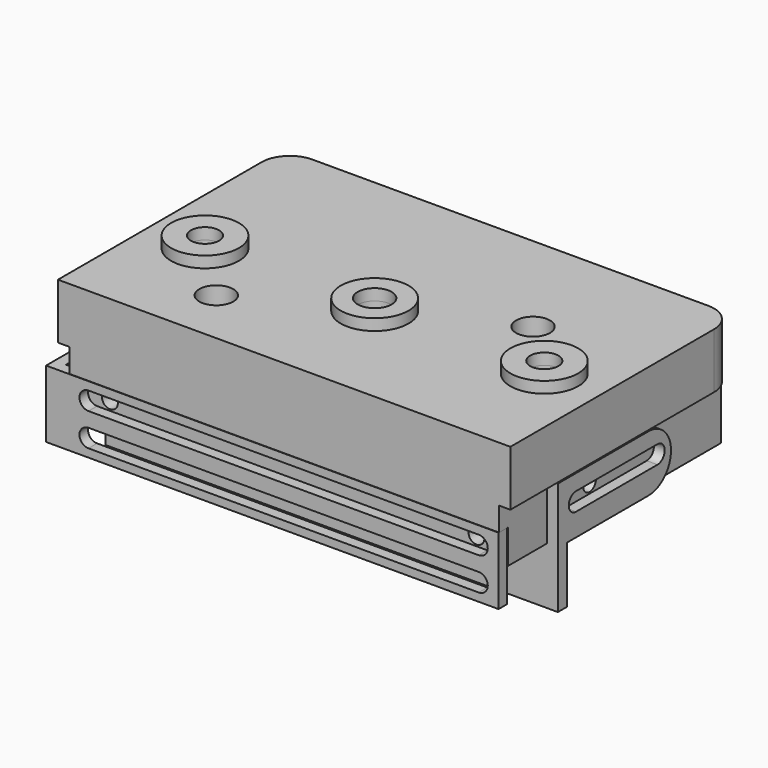
from build123d import *

# Parameters (mm, degrees)
F0_W          = 80
F0_H          = 50
F0_R          = 3
F0_R_2        = 5.1
F1_DEPTH      = 20
F3_DEPTH      = 20
F4_R          = 5
F4_R_2        = 2.5
F5_DEPTH      = 20
F5_DEPTH_BACK = 2
F4_R_3        = 3
F6_R          = 6
F6_R_2        = 5.1
F6_R_3        = 4.2549241369
F7_DEPTH      = 2
F6_R_4        = 3.9454924111
F6_R_5        = 4.3855625848
F8_W          = 80
F8_H          = 2
F9_DEPTH      = 10
F10_W         = 2
F10_H         = 50
F11_DEPTH     = 10.2
F12_W         = 1.9
F12_H         = 25
F13_DEPTH     = 10
F15_DEPTH     = 90
F16_R         = 4.99999
F17_R         = 1.4
F18_R         = 1.4
F19_DEPTH     = 2.5
F20_R         = 5
F21_W         = 2
F21_H         = 6
F22_DEPTH     = 80
F24_START     = 0.1
F23_W         = 12.5
F23_H         = 5.95
F23_W_2       = 10.5
F23_H_2       = 11.9
F24_DEPTH     = 2
F25_W         = 1.9
F25_H         = 11.9
F26_DEPTH     = 80
F27_W         = 9
F27_H         = 3
F28_DEPTH     = 25
F29_R         = 2
F31_DEPTH     = 25
F32_R         = 1.4
F33_DEPTH     = 5


# Not quite as in the source:
# - a fillet or chamfer is up to 0.001 mm smaller than in the source, because OpenCascade refuses the exact size
# - a feature names something its author has since deleted; it is built from what else it names


with BuildPart() as f1:
    # F0 (on Top) → F1 (new body)
    with BuildSketch(Plane.XY):
        Rectangle(F0_W, F0_H)
        with Locations((-20, -15)):
            Circle(F0_R, mode=Mode.SUBTRACT)
        with Locations((-30, -5)):
            Circle(F0_R_2, mode=Mode.SUBTRACT)
        with Locations((0, -5)):
            Circle(F0_R_2, mode=Mode.SUBTRACT)
        with Locations((30, -5)):
            Circle(F0_R_2, mode=Mode.SUBTRACT)
        with Locations((20, 5)):
            Circle(F0_R, mode=Mode.SUBTRACT)
    extrude(amount=F1_DEPTH)

    # F2 (on face) → F3 (cut)
    with BuildSketch(Plane(origin=(0, 25, 0), x_dir=(-1, 0, 0), z_dir=(0, 1, 0))):
        with BuildLine():
            Line((-3, 15), (3, 15))
            ThreePointArc((3, 15), (0, 18), (-3, 15))
        make_face()
        with BuildLine():
            ThreePointArc((-3, 15), (0, 12), (3, 15))
            Line((3, 15), (-3, 15))
        make_face()
        with BuildLine():
            Line((-32.5, 15), (-27.5, 15))
            ThreePointArc((-27.5, 15), (-30, 17.5), (-32.5, 15))
        make_face()
        with BuildLine():
            ThreePointArc((-32.5, 15), (-30, 12.5), (-27.5, 15))
            Line((-27.5, 15), (-32.5, 15))
        make_face()
        with BuildLine():
            ThreePointArc((32.5, 15), (30, 17.5), (27.5, 15))
            Line((27.5, 15), (32.5, 15))
        make_face()
        with BuildLine():
            Line((32.5, 15), (27.5, 15))
            ThreePointArc((27.5, 15), (30, 12.5), (32.5, 15))
        make_face()
        with BuildLine():
            Line((-3, 0), (3, 0))
            Line((3, 0), (3, 15))
            ThreePointArc((3, 15), (0, 12), (-3, 15))
            Line((-3, 15), (-3, 0))
        make_face()
        with BuildLine():
            Line((-32.5, 0), (-27.5, 0))
            Line((-27.5, 0), (-27.5, 15))
            ThreePointArc((-27.5, 15), (-30, 12.5), (-32.5, 15))
            Line((-32.5, 15), (-32.5, 0))
        make_face()
        with BuildLine():
            Line((27.5, 15), (27.5, 0))
            Line((27.5, 0), (32.5, 0))
            Line((32.5, 0), (32.5, 15))
            ThreePointArc((32.5, 15), (30, 12.5), (27.5, 15))
        make_face()
    extrude(amount=-F3_DEPTH, mode=Mode.SUBTRACT)

    # F10 (on face) → F11 (cut)
    with BuildSketch(Plane(origin=(0, 0, 0), x_dir=(1, 0, 0), z_dir=(0, 0, -1))):
        with Locations((-39, 0)):
            Rectangle(F10_W, F10_H)
        with Locations((39, 0)):
            Rectangle(F10_W, F10_H)
    extrude(amount=-F11_DEPTH, mode=Mode.SUBTRACT)

    # F17 (on face) + F18 (on face) → F19 (cut, symmetric)
    with BuildSketch(Plane(origin=(-38, 0, 0), x_dir=(0, -1, 0), z_dir=(-1, 0, 0))):
        with Locations((5, 5.6)):
            Circle(F17_R)
    with BuildSketch(Plane.YZ.offset(38)):
        with Locations((-5, 5.6)):
            Circle(F18_R)
    extrude(amount=F19_DEPTH, both=True, dir=(-1, 0, 0), mode=Mode.SUBTRACT)

    # F20
    f20_edges = [f1.edges().sort_by_distance(p)[0] for p in [
        (-40, 25, 15.1),
        (40, 25, 15.1),
    ]]
    fillet(f20_edges, radius=F20_R)

    # F21 (on face) → F22 (cut)
    with BuildSketch(Plane(origin=(-38, 0, 0), x_dir=(0, -1, 0), z_dir=(-1, 0, 0))):
        with Locations((24, 3)):
            Rectangle(F21_W, F21_H)
    extrude(amount=-F22_DEPTH, mode=Mode.SUBTRACT)

    # F32 (on face) → F33 (cut)
    with BuildSketch(Plane.XZ.offset(23)):
        with Locations((-32.4034833738, 2.9)):
            Circle(F32_R)
        with Locations((32.4034833738, 2.9)):
            Circle(F32_R)
    extrude(amount=-F33_DEPTH, mode=Mode.SUBTRACT)


with BuildPart() as f5:
    # F4 (on face) → F5 (new body, two sides)
    with BuildSketch(Plane.XY.offset(20)) as f5_sk:
        with Locations((30, -5)):
            Circle(F4_R)
        with Locations((30, -5)):
            Circle(F4_R_2, mode=Mode.SUBTRACT)
    extrude(amount=-F5_DEPTH)
    extrude(f5_sk.sketch, amount=F5_DEPTH_BACK)

    # F6 (on face) → F7, piece 3 (join)
    with BuildSketch(Plane.XY.offset(20)):
        with Locations((30, -5)):
            Circle(F6_R)
        with Locations((30, -5)):
            Circle(F6_R_2, mode=Mode.SUBTRACT)
        with Locations((30, -5)):
            Circle(F6_R_2)
        with Locations((30, -5)):
            Circle(F6_R_5, mode=Mode.SUBTRACT)
    extrude(amount=F7_DEPTH)


with BuildPart() as f5b:
    # F4 (on face) → F5, piece 2 (new body, two sides)
    with BuildSketch(Plane.XY.offset(20)) as f5_2_sk:
        with Locations((0, -5)):
            Circle(F4_R)
        with Locations((0, -5)):
            Circle(F4_R_3, mode=Mode.SUBTRACT)
    extrude(amount=-F5_DEPTH)
    extrude(f5_2_sk.sketch, amount=F5_DEPTH_BACK)

    # F6 (on face) → F7 (join)
    with BuildSketch(Plane.XY.offset(20)):
        with Locations((0, -5)):
            Circle(F6_R)
        with Locations((0, -5)):
            Circle(F6_R_2, mode=Mode.SUBTRACT)
        with Locations((0, -5)):
            Circle(F6_R_2)
        with Locations((0, -5)):
            Circle(F6_R_3, mode=Mode.SUBTRACT)
    extrude(amount=F7_DEPTH)


with BuildPart() as f5c:
    # F4 (on face) → F5, piece 3 (new body, two sides)
    with BuildSketch(Plane.XY.offset(20)) as f5_3_sk:
        with Locations((-30, -5)):
            Circle(F4_R)
        with Locations((-30, -5)):
            Circle(F4_R_2, mode=Mode.SUBTRACT)
    extrude(amount=-F5_DEPTH)
    extrude(f5_3_sk.sketch, amount=F5_DEPTH_BACK)

    # F6 (on face) → F7, piece 2 (join)
    with BuildSketch(Plane.XY.offset(20)):
        with Locations((-30, -5)):
            Circle(F6_R)
        with Locations((-30, -5)):
            Circle(F6_R_2, mode=Mode.SUBTRACT)
        with Locations((-30, -5)):
            Circle(F6_R_2)
        with Locations((-30, -5)):
            Circle(F6_R_4, mode=Mode.SUBTRACT)
    extrude(amount=F7_DEPTH)


with BuildPart() as f9:
    # F8 (on face) → F9 (new body)
    with BuildSketch(Plane(origin=(0, 0, 0), x_dir=(1, 0, 0), z_dir=(0, 0, -1))):
        with Locations((0, 13.5)):
            Rectangle(F8_W, F8_H)
    extrude(amount=F9_DEPTH)

    # F12 (on face) → F13 (join)
    with BuildSketch(Plane(origin=(0, 0, 0), x_dir=(1, 0, 0), z_dir=(0, 0, -1))):
        with Locations((-39.05, 2)):
            Rectangle(F12_W, F12_H)
        with Locations((39.05, 2)):
            Rectangle(F12_W, F12_H)
    extrude(amount=-F13_DEPTH)

    # F14 (on face) → F15 (cut)
    with BuildSketch(Plane(origin=(-40, 0, 0), x_dir=(0, -1, 0), z_dir=(-1, 0, 0))):
        with BuildLine():
            ThreePointArc((-5.9, 5.6), (-6.3686291501, 6.7313708499), (-7.5, 7.2))
            Line((-7.5, 7.2), (-7.5, 4))
            ThreePointArc((-7.5, 4), (-6.3686291501, 4.4686291501), (-5.9, 5.6))
        make_face()
        with BuildLine():
            Line((10.5, 7.2), (-7.5, 7.2))
            ThreePointArc((-7.5, 7.2), (-6.3686291501, 6.7313708499), (-5.9, 5.6))
            ThreePointArc((-5.9, 5.6), (-6.3686291501, 4.4686291501), (-7.5, 4))
            Line((-7.5, 4), (10.5, 4))
            ThreePointArc((10.5, 4), (8.9, 5.6), (10.5, 7.2))
        make_face()
        with BuildLine():
            Line((-7.5, 4), (-7.5, 7.2))
            ThreePointArc((-7.5, 7.2), (-9.1, 5.6), (-7.5, 4))
        make_face()
        with BuildLine():
            ThreePointArc((12.1, 5.6), (11.6313708499, 6.7313708499), (10.5, 7.2))
            Line((10.5, 7.2), (10.5, 4))
            ThreePointArc((10.5, 4), (11.6313708499, 4.4686291501), (12.1, 5.6))
        make_face()
        with BuildLine():
            Line((10.5, 4), (10.5, 7.2))
            ThreePointArc((10.5, 7.2), (8.9, 5.6), (10.5, 4))
        make_face()
    extrude(amount=-F15_DEPTH, mode=Mode.SUBTRACT)

    # F16 (radius 5 in the source; OpenCascade refuses exactly that, so slightly less here)
    f16_edges = [f9.edges().sort_by_distance(p)[0] for p in [
        (-39.05, 10.5, 10),
        (-39.05, 10.5, 0),
        (39.05, 10.5, 10),
        (39.05, 10.5, 0),
    ]]
    fillet(f16_edges, radius=F16_R)


with BuildPart() as f24:
    # F23 (on face) → F24 (new body)
    with BuildSketch(Plane(origin=(-40, 0, 0), x_dir=(0, -1, 0), z_dir=(-1, 0, 0)).offset(F24_START)):
        with Locations((6.25, -2.975)):
            Rectangle(F23_W, F23_H)
        with Locations((19.75, 0)):
            Rectangle(F23_W_2, F23_H_2)
        with BuildLine():
            Line((12.5, -5.95), (14.5, -5.95))
            Line((14.5, -5.95), (14.5, 5.95))
            Line((14.5, 5.95), (12.0612494996, 5.95))
            ThreePointArc((12.0612494996, 5.95), (11.7489995997, 4.6), (10.5, 4))
            Line((10.5, 4), (0, 4))
            Line((0, 4), (0, 0))
            Line((0, 0), (12.5, 0))
            Line((12.5, 0), (12.5, -5.95))
        make_face()
        with BuildLine():
            ThreePointArc((10.5, 4), (11.7489995997, 4.6), (12.0612494996, 5.95))
            Line((12.0612494996, 5.95), (0, 5.95))
            Line((0, 5.95), (0, 4))
            Line((0, 4), (10.5, 4))
        make_face()
    extrude(amount=F24_DEPTH)

    # F25 (on face) → F26 (join)
    with BuildSketch(Plane(origin=(-42.1, 0, 0), x_dir=(0, -1, 0), z_dir=(-1, 0, 0))):
        with Locations((24.05, 0)):
            Rectangle(F25_W, F25_H)
    extrude(amount=-F26_DEPTH)

    # F27 (on face) → F28 (cut)
    with BuildSketch(Plane(origin=(-42.1, 0, 0), x_dir=(0, -1, 0), z_dir=(-1, 0, 0))):
        with Locations((4.5, 4.45)):
            Rectangle(F27_W, F27_H)
        with Locations((4.5, -4.45)):
            Rectangle(F27_W, F27_H)
    extrude(amount=-F28_DEPTH, mode=Mode.SUBTRACT)

    # F29
    f29_edges = [f24.edges().sort_by_distance(p)[0] for p in [
        (-41.1, -9, 2.95),
        (-41.1, -9, -2.95),
    ]]
    fillet(f29_edges, radius=F29_R)

    # F30 (on face) → F31 (cut)
    with BuildSketch(Plane.XZ.offset(25)):
        with BuildLine():
            Line((34.4, 4.5), (-34.6, 4.5))
            ThreePointArc((-34.6, 4.5), (-33.4686291501, 4.0313708499), (-33, 2.9))
            ThreePointArc((-33, 2.9), (-33.4686291501, 1.7686291501), (-34.6, 1.3))
            Line((-34.6, 1.3), (34.4, 1.3))
            ThreePointArc((34.4, 1.3), (32.8, 2.9), (34.4, 4.5))
        make_face()
        with BuildLine():
            ThreePointArc((-33, 2.9), (-33.4686291501, 4.0313708499), (-34.6, 4.5))
            Line((-34.6, 4.5), (-34.6, 1.3))
            ThreePointArc((-34.6, 1.3), (-33.4686291501, 1.7686291501), (-33, 2.9))
        make_face()
        with BuildLine():
            Line((-34.6, 1.3), (-34.6, 4.5))
            ThreePointArc((-34.6, 4.5), (-36.2, 2.9), (-34.6, 1.3))
        make_face()
        with BuildLine():
            ThreePointArc((-33, -2.9), (-33.4686291501, -1.7686291501), (-34.6, -1.3))
            ThreePointArc((-34.6, -1.3), (-36.2, -2.9), (-34.6, -4.5))
            ThreePointArc((-34.6, -4.5), (-33.4686291501, -4.0313708499), (-33, -2.9))
        make_face()
        with BuildLine():
            Line((34.4, -1.3), (-34.6, -1.3))
            ThreePointArc((-34.6, -1.3), (-33.4686291501, -1.7686291501), (-33, -2.9))
            ThreePointArc((-33, -2.9), (-33.4686291501, -4.0313708499), (-34.6, -4.5))
            Line((-34.6, -4.5), (34.4, -4.5))
            ThreePointArc((34.4, -4.5), (32.8, -2.9), (34.4, -1.3))
        make_face()
        with BuildLine():
            ThreePointArc((36, -2.9), (35.5313708499, -1.7686291501), (34.4, -1.3))
            ThreePointArc((34.4, -1.3), (32.8, -2.9), (34.4, -4.5))
            ThreePointArc((34.4, -4.5), (35.5313708499, -4.0313708499), (36, -2.9))
        make_face()
        with BuildLine():
            ThreePointArc((36, 2.9), (35.5313708499, 4.0313708499), (34.4, 4.5))
            Line((34.4, 4.5), (34.4, 1.3))
            ThreePointArc((34.4, 1.3), (35.5313708499, 1.7686291501), (36, 2.9))
        make_face()
        with BuildLine():
            Line((34.4, 1.3), (34.4, 4.5))
            ThreePointArc((34.4, 4.5), (32.8, 2.9), (34.4, 1.3))
        make_face()
    extrude(amount=-F31_DEPTH, mode=Mode.SUBTRACT)


solid = Compound([f1.part, f5.part, f5b.part, f5c.part, f9.part, f24.part])
